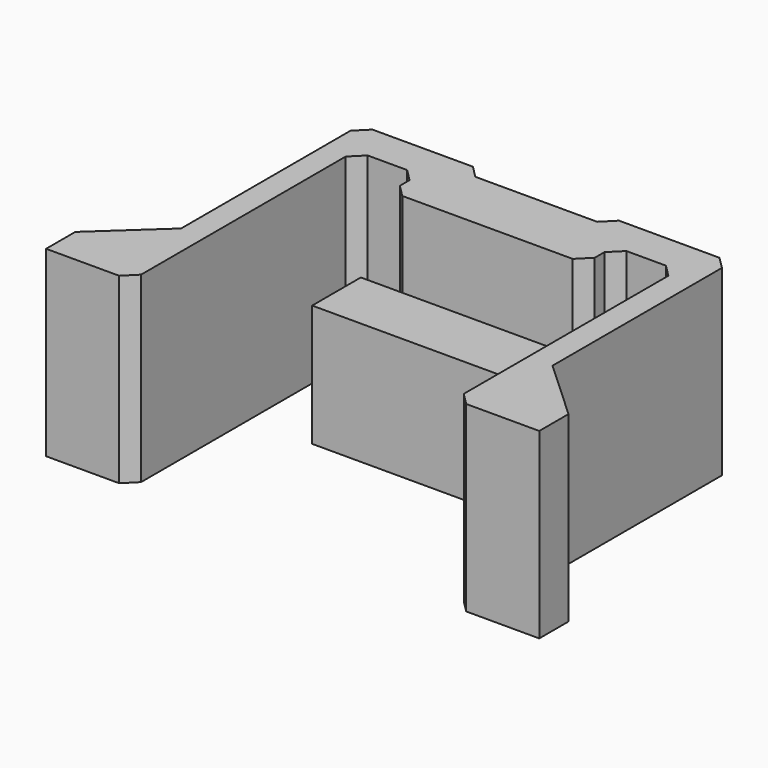
from build123d import *

# Parameters (mm, degrees)
F0_W     = 16
F0_H     = 3
F1_DEPTH = 15
F2_SIZE  = 0.99999
F0_H_2   = 5
F3_DEPTH = 10


# Not quite as in the source:
# - a fillet or chamfer is up to 0.001 mm smaller than in the source, because OpenCascade refuses the exact size


with BuildPart() as f1:
    # F0 (on Top) → F1 (new body)
    with BuildSketch(Plane.XY):
        Polygon((-15.25, 7.6134982519), (-15.25, 0), (-13.25, 0), (-13.25, 23), (-8, 23), (8, 23), (13.25, 23), (13.25, 0), (15.25, 0), (15.25, 7.6134982519), (15.25, 26), (5, 26), (5, 25), (-5, 25), (-5, 26), (-15.25, 26), align=None)
        with Locations((0, 21.5)):
            Rectangle(F0_W, F0_H)
        Polygon((15.25, 7.6134982519), (15.25, 0), (20.25, 0), (20.25, 3), align=None)
        Polygon((-20.25, 0), (-15.25, 0), (-15.25, 7.6134982519), (-20.25, 3), align=None)
    extrude(amount=F1_DEPTH)

    # F2 (size 1 in the source; OpenCascade refuses exactly that, so slightly less here)
    f2_edges = [f1.edges().sort_by_distance(p)[0] for p in [
        (-13.25, 23, 7.5),
        (13.25, 23, 7.5),
        (15.25, 26, 7.5),
        (-15.25, 26, 7.5),
        (-5, 26, 7.5),
        (5, 26, 7.5),
        (-8, 23, 7.5),
        (-8, 20, 7.5),
        (8, 23, 7.5),
        (8, 20, 7.5),
        (13.25, 0, 7.5),
        (-13.25, 0, 7.5),
    ]]
    chamfer(f2_edges, length=F2_SIZE)


with BuildPart() as f3:
    # F0 (on Top) → F3 (new body)
    with BuildSketch(Plane.XY):
        with Locations((0, 14.5)):
            Rectangle(F0_W, F0_H_2)
    extrude(amount=F3_DEPTH)


solid = Compound([f1.part, f3.part])
